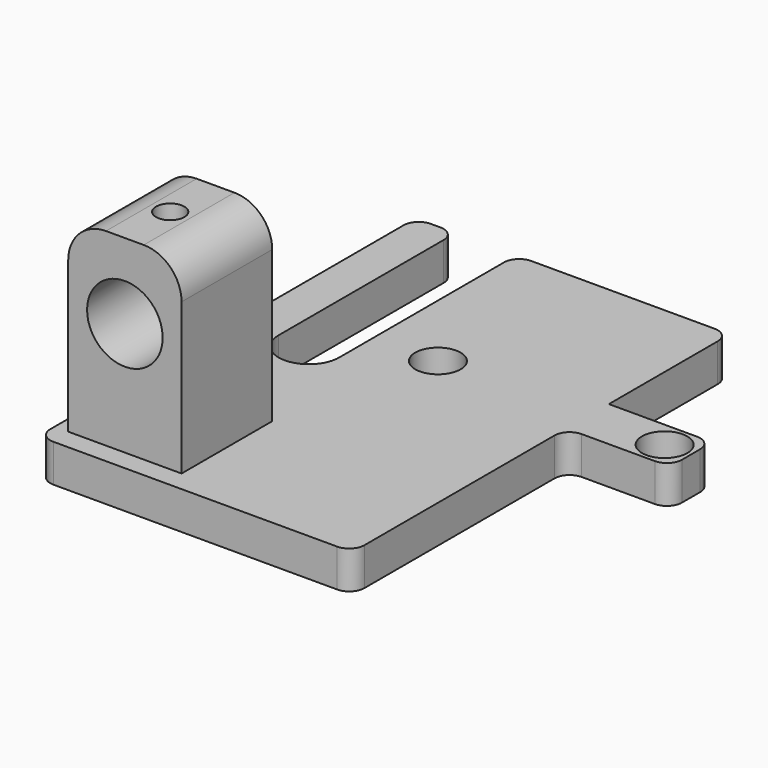
from build123d import *

# Parameters (mm, degrees)
F0_R      = 1.7
F0_W      = 23.3248192817
F0_H      = 35.4459092319
F0_H_2    = 20
F1_DEPTH  = 5
F2_R      = 3
F2_R_2    = 1.7
F3_DEPTH  = 4
F4_W      = 15
F4_H      = 15
F5_DEPTH  = 25
F6_R      = 5
F7_DEPTH  = 15
F8_R      = 2
F9_R      = 1.875
F10_DEPTH = 7
F11_R     = 5


with BuildPart() as f1:
    # F0 (on Top) → F1 (new body)
    with BuildSketch(Plane.XY):
        Polygon((23.3248192817, 0), (0, 0), (0, -7), (23.3248192817, -7), (37, -7), (37, 0), align=None)
        with Locations((3.5, -3.5)):
            Circle(F0_R, mode=Mode.SUBTRACT)
        with Locations((33.5, -3.5)):
            Circle(F0_R, mode=Mode.SUBTRACT)
        with Locations((11.6624096408, -24.722954616)):
            Rectangle(F0_W, F0_H)
        with Locations((11.6624096408, 10)):
            Rectangle(F0_W, F0_H_2)
        with BuildLine():
            Line((0, -7), (0, 0))
            Line((0, 0), (0, 20))
            Line((0, 20), (-4.9525605589, 20))
            Line((-4.9525605589, 20), (-4.9525605589, -9.2811752111))
            ThreePointArc((-4.9525605589, -9.2811752111), (-8.9525605589, -13.2811752111), (-12.9525605589, -9.2811752111))
            Line((-12.9525605589, -9.2811752111), (-12.9525605589, 20))
            Line((-12.9525605589, 20), (-18.2450078428, 20))
            Line((-18.2450078428, 20), (-18.2450078428, -42.4459092319))
            Line((-18.2450078428, -42.4459092319), (0, -42.4459092319))
            Line((0, -42.4459092319), (0, -7))
        make_face()
    extrude(amount=F1_DEPTH)

    # F2 (on face) → F3 (cut)
    with BuildSketch(Plane.XY.offset(5)):
        with Locations((3.5, -3.5)):
            Circle(F2_R)
        with Locations((3.5, -3.5)):
            Circle(F2_R_2, mode=Mode.SUBTRACT)
        with Locations((33.5, -3.5)):
            Circle(F2_R)
        with Locations((33.5, -3.5)):
            Circle(F2_R_2, mode=Mode.SUBTRACT)
    extrude(amount=-F3_DEPTH, mode=Mode.SUBTRACT)

    # F4 (on face) → F5 (join)
    with BuildSketch(Plane.XY.offset(5)):
        with Locations((-8.9525605589, -32.2227959335)):
            Rectangle(F4_W, F4_H)
    extrude(amount=F5_DEPTH)

    # F6 (on face) → F7 (cut)
    with BuildSketch(Plane(origin=(0, -24.7227959335, 0), x_dir=(-1, 0, 0), z_dir=(0, 1, 0))):
        with Locations((8.9525605589, 20)):
            Circle(F6_R)
    extrude(amount=-F7_DEPTH, mode=Mode.SUBTRACT)

    # F8
    f8_edges = [f1.edges().sort_by_distance(p)[0] for p in [
        (23.324819, 20, 2.5),
        (37, 0, 2.5),
        (37, -7, 2.5),
        (23.324819, -42.445909, 2.5),
        (-18.245008, 20, 2.5),
        (-18.245008, -42.445909, 2.5),
        (23.324819, -7, 2.5),
        (-4.952561, 20, 2.5),
        (-12.952561, 20, 2.5),
    ]]
    fillet(f8_edges, radius=F8_R)

    # F9 (on face) → F10 (cut)
    with BuildSketch(Plane.XY.offset(30)):
        with Locations((-8.9525605589, -32.2227959335)):
            Circle(F9_R)
    extrude(amount=-F10_DEPTH, mode=Mode.SUBTRACT)

    # F11
    f11_edges = [f1.edges().sort_by_distance(p)[0] for p in [
        (-1.452561, -32.222796, 30),
        (-16.452561, -32.222796, 30),
    ]]
    fillet(f11_edges, radius=F11_R)


solid = f1.part
